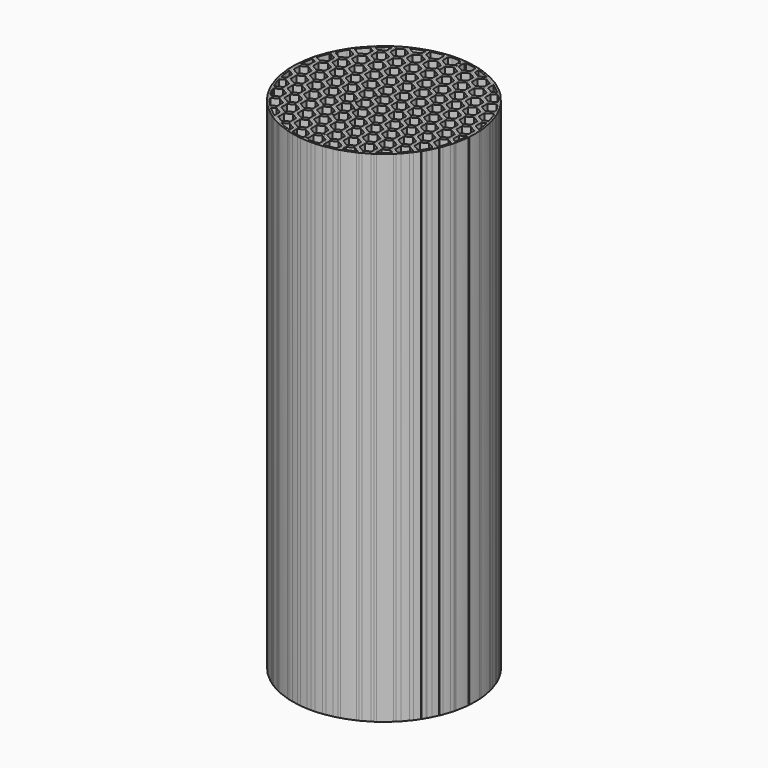
from build123d import *

# Parameters (mm, degrees)
F1_DEPTH  = 130
F0_R      = 23.75
F0_R_2    = 23.25
F14_R     = 45.818739932
F14_R_2   = 23.75
F15_DEPTH = 130


with BuildPart() as f1:
    # F0 (on Top) → F1 (new body)
    with BuildSketch(Plane.XY):
        Polygon((2.1135, -1.2202297939), (2.1135, 1.2202297939), (0, 2.4404595879), (-2.1135, 1.2202297939), (-2.1135, -1.2202297939), (0, -2.4404595879), align=None)
        Polygon((0, 1.8631093187), (1.6135, 0.9315546593), (1.6135, -0.9315546593), (0, -1.8631093187), (-1.6135, -0.9315546593), (-1.6135, 0.9315546593), align=None, mode=Mode.SUBTRACT)
    extrude(amount=F1_DEPTH)


with BuildPart() as f1b:
    # F0 (on Top) → F1, piece 2 (new body)
    with BuildSketch(Plane.XY):
        Circle(F0_R)
        Circle(F0_R_2, mode=Mode.SUBTRACT)
    extrude(amount=F1_DEPTH)


with BuildPart() as f3_1:
    # F3: copy of F1
    add(f1.part.moved(Location((4.227, 0, 0))))


with BuildPart() as f4_1:
    # F4: copy of F1
    add(f1.part.moved(Location((8.454, 0, 0))))


with BuildPart() as f4_2:
    # F4: copy of F3_1
    add(f3_1.part.moved(Location((8.454, 0, 0))))


with BuildPart() as f5_1:
    # F5: copy of F4_1
    add(f4_1.part.moved(Location((8.454, 0, 0))))


with BuildPart() as f5_2:
    # F5: copy of F4_2
    add(f4_2.part.moved(Location((8.454, 0, 0))))


with BuildPart() as f6_1:
    # F6: copy of F1
    add(f1.part.moved(Location((2.1135, 3.65, 0))))


with BuildPart() as f6_2:
    # F6: copy of F3_1
    add(f3_1.part.moved(Location((2.1135, 3.65, 0))))


with BuildPart() as f6_3:
    # F6: copy of F4_1
    add(f4_1.part.moved(Location((2.1135, 3.65, 0))))


with BuildPart() as f6_4:
    # F6: copy of F4_2
    add(f4_2.part.moved(Location((2.1135, 3.65, 0))))


with BuildPart() as f6_5:
    # F6: copy of F5_1
    add(f5_1.part.moved(Location((2.1135, 3.65, 0))))


with BuildPart() as f6_6:
    # F6: copy of F5_2
    add(f5_2.part.moved(Location((2.1135, 3.65, 0))))


with BuildPart() as f7_1:
    # F7: copy of F6_1
    add(f6_1.part.moved(Location((4.228, 7.3, 0))))


with BuildPart() as f7_2:
    # F7: copy of F1
    add(f1.part.moved(Location((4.228, 7.3, 0))))


with BuildPart() as f7_3:
    # F7: copy of F3_1
    add(f3_1.part.moved(Location((4.228, 7.3, 0))))


with BuildPart() as f7_4:
    # F7: copy of F6_2
    add(f6_2.part.moved(Location((4.228, 7.3, 0))))


with BuildPart() as f7_5:
    # F7: copy of F6_3
    add(f6_3.part.moved(Location((4.228, 7.3, 0))))


with BuildPart() as f7_6:
    # F7: copy of F4_1
    add(f4_1.part.moved(Location((4.228, 7.3, 0))))


with BuildPart() as f7_7:
    # F7: copy of F4_2
    add(f4_2.part.moved(Location((4.228, 7.3, 0))))


with BuildPart() as f7_8:
    # F7: copy of F6_4
    add(f6_4.part.moved(Location((4.228, 7.3, 0))))


with BuildPart() as f7_9:
    # F7: copy of F6_5
    add(f6_5.part.moved(Location((4.228, 7.3, 0))))


with BuildPart() as f7_10:
    # F7: copy of F5_1
    add(f5_1.part.moved(Location((4.228, 7.3, 0))))


with BuildPart() as f7_11:
    # F7: copy of F6_6
    add(f6_6.part.moved(Location((4.228, 7.3, 0))))


with BuildPart() as f7_12:
    # F7: copy of F5_2
    add(f5_2.part.moved(Location((4.228, 7.3, 0))))


with BuildPart() as f8_1:
    # F8: copy of F1
    add(f1.part.moved(Location((-4.228, -14.6, 0))))


with BuildPart() as f8_2:
    # F8: copy of F7_4
    add(f7_4.part.moved(Location((-4.228, -14.6, 0))))


with BuildPart() as f8_3:
    # F8: copy of F7_1
    add(f7_1.part.moved(Location((-4.228, -14.6, 0))))


with BuildPart() as f8_4:
    # F8: copy of F7_6
    add(f7_6.part.moved(Location((-4.228, -14.6, 0))))


with BuildPart() as f8_5:
    # F8: copy of F7_3
    add(f7_3.part.moved(Location((-4.228, -14.6, 0))))


with BuildPart() as f8_6:
    # F8: copy of F7_2
    add(f7_2.part.moved(Location((-4.228, -14.6, 0))))


with BuildPart() as f8_7:
    # F8: copy of F6_3
    add(f6_3.part.moved(Location((-4.228, -14.6, 0))))


with BuildPart() as f8_8:
    # F8: copy of F6_2
    add(f6_2.part.moved(Location((-4.228, -14.6, 0))))


with BuildPart() as f8_9:
    # F8: copy of F6_1
    add(f6_1.part.moved(Location((-4.228, -14.6, 0))))


with BuildPart() as f8_10:
    # F8: copy of F4_2
    add(f4_2.part.moved(Location((-4.228, -14.6, 0))))


with BuildPart() as f8_11:
    # F8: copy of F4_1
    add(f4_1.part.moved(Location((-4.228, -14.6, 0))))


with BuildPart() as f8_12:
    # F8: copy of F3_1
    add(f3_1.part.moved(Location((-4.228, -14.6, 0))))


with BuildPart() as f8_13:
    # F8: copy of F6_4
    add(f6_4.part.moved(Location((-4.228, -14.6, 0))))


with BuildPart() as f8_14:
    # F8: copy of F7_7
    add(f7_7.part.moved(Location((-4.228, -14.6, 0))))


with BuildPart() as f8_15:
    # F8: copy of F7_5
    add(f7_5.part.moved(Location((-4.228, -14.6, 0))))


with BuildPart() as f8_16:
    # F8: copy of F7_8
    add(f7_8.part.moved(Location((-4.228, -14.6, 0))))


with BuildPart() as f8_17:
    # F8: copy of F7_10
    add(f7_10.part.moved(Location((-4.228, -14.6, 0))))


with BuildPart() as f8_18:
    # F8: copy of F6_5
    add(f6_5.part.moved(Location((-4.228, -14.6, 0))))


with BuildPart() as f8_19:
    # F8: copy of F5_1
    add(f5_1.part.moved(Location((-4.228, -14.6, 0))))


with BuildPart() as f8_20:
    # F8: copy of F5_2
    add(f5_2.part.moved(Location((-4.228, -14.6, 0))))


with BuildPart() as f8_21:
    # F8: copy of F6_6
    add(f6_6.part.moved(Location((-4.228, -14.6, 0))))


with BuildPart() as f8_22:
    # F8: copy of F7_12
    add(f7_12.part.moved(Location((-4.228, -14.6, 0))))


with BuildPart() as f8_23:
    # F8: copy of F7_9
    add(f7_9.part.moved(Location((-4.228, -14.6, 0))))


with BuildPart() as f9_1:
    # F9: copy of F8_9
    add(f8_9.part.moved(Location((-25.369, 0, 0))))


with BuildPart() as f9_2:
    # F9: copy of F1
    add(f1.part.moved(Location((-25.369, 0, 0))))


with BuildPart() as f9_3:
    # F9: copy of F8_8
    add(f8_8.part.moved(Location((-25.369, 0, 0))))


with BuildPart() as f9_4:
    # F9: copy of F8_4
    add(f8_4.part.moved(Location((-25.369, 0, 0))))


with BuildPart() as f9_5:
    # F9: copy of F7_4
    add(f7_4.part.moved(Location((-25.369, 0, 0))))


with BuildPart() as f9_6:
    # F9: copy of F8_5
    add(f8_5.part.moved(Location((-25.369, 0, 0))))


with BuildPart() as f9_7:
    # F9: copy of F8_13
    add(f8_13.part.moved(Location((-25.369, 0, 0))))


with BuildPart() as f9_8:
    # F9: copy of F8_6
    add(f8_6.part.moved(Location((-25.369, 0, 0))))


with BuildPart() as f9_9:
    # F9: copy of F8_3
    add(f8_3.part.moved(Location((-25.369, 0, 0))))


with BuildPart() as f9_10:
    # F9: copy of F7_1
    add(f7_1.part.moved(Location((-25.369, 0, 0))))


with BuildPart() as f9_11:
    # F9: copy of F7_3
    add(f7_3.part.moved(Location((-25.369, 0, 0))))


with BuildPart() as f9_12:
    # F9: copy of F7_2
    add(f7_2.part.moved(Location((-25.369, 0, 0))))


with BuildPart() as f9_13:
    # F9: copy of F6_3
    add(f6_3.part.moved(Location((-25.369, 0, 0))))


with BuildPart() as f9_14:
    # F9: copy of F6_2
    add(f6_2.part.moved(Location((-25.369, 0, 0))))


with BuildPart() as f9_15:
    # F9: copy of F6_1
    add(f6_1.part.moved(Location((-25.369, 0, 0))))


with BuildPart() as f9_16:
    # F9: copy of F4_1
    add(f4_1.part.moved(Location((-25.369, 0, 0))))


with BuildPart() as f9_17:
    # F9: copy of F3_1
    add(f3_1.part.moved(Location((-25.369, 0, 0))))


with BuildPart() as f9_18:
    # F9: copy of F8_2
    add(f8_2.part.moved(Location((-25.369, 0, 0))))


with BuildPart() as f9_19:
    # F9: copy of F8_7
    add(f8_7.part.moved(Location((-25.369, 0, 0))))


with BuildPart() as f9_20:
    # F9: copy of F8_15
    add(f8_15.part.moved(Location((-25.369, 0, 0))))


with BuildPart() as f9_21:
    # F9: copy of F8_1
    add(f8_1.part.moved(Location((-25.369, 0, 0))))


with BuildPart() as f9_22:
    # F9: copy of F8_12
    add(f8_12.part.moved(Location((-25.369, 0, 0))))


with BuildPart() as f9_23:
    # F9: copy of F8_11
    add(f8_11.part.moved(Location((-25.369, 0, 0))))


with BuildPart() as f9_24:
    # F9: copy of F8_10
    add(f8_10.part.moved(Location((-25.369, 0, 0))))


with BuildPart() as f9_25:
    # F9: copy of F8_20
    add(f8_20.part.moved(Location((-25.369, 0, 0))))


with BuildPart() as f9_26:
    # F9: copy of F7_11
    add(f7_11.part.moved(Location((-25.369, 0, 0))))


with BuildPart() as f9_27:
    # F9: copy of F8_14
    add(f8_14.part.moved(Location((-25.369, 0, 0))))


with BuildPart() as f9_28:
    # F9: copy of F7_5
    add(f7_5.part.moved(Location((-25.369, 0, 0))))


with BuildPart() as f9_29:
    # F9: copy of F7_8
    add(f7_8.part.moved(Location((-25.369, 0, 0))))


with BuildPart() as f9_30:
    # F9: copy of F7_9
    add(f7_9.part.moved(Location((-25.369, 0, 0))))


with BuildPart() as f9_31:
    # F9: copy of F8_21
    add(f8_21.part.moved(Location((-25.369, 0, 0))))


with BuildPart() as f9_32:
    # F9: copy of F7_10
    add(f7_10.part.moved(Location((-25.369, 0, 0))))


with BuildPart() as f9_33:
    # F9: copy of F7_7
    add(f7_7.part.moved(Location((-25.369, 0, 0))))


with BuildPart() as f9_34:
    # F9: copy of F8_19
    add(f8_19.part.moved(Location((-25.369, 0, 0))))


with BuildPart() as f9_35:
    # F9: copy of F7_12
    add(f7_12.part.moved(Location((-25.369, 0, 0))))


with BuildPart() as f9_36:
    # F9: copy of F7_6
    add(f7_6.part.moved(Location((-25.369, 0, 0))))


with BuildPart() as f9_37:
    # F9: copy of F6_4
    add(f6_4.part.moved(Location((-25.369, 0, 0))))


with BuildPart() as f9_38:
    # F9: copy of F6_5
    add(f6_5.part.moved(Location((-25.369, 0, 0))))


with BuildPart() as f9_39:
    # F9: copy of F6_6
    add(f6_6.part.moved(Location((-25.369, 0, 0))))


with BuildPart() as f9_40:
    # F9: copy of F4_2
    add(f4_2.part.moved(Location((-25.369, 0, 0))))


with BuildPart() as f9_41:
    # F9: copy of F5_2
    add(f5_2.part.moved(Location((-25.369, 0, 0))))


with BuildPart() as f9_42:
    # F9: copy of F5_1
    add(f5_1.part.moved(Location((-25.369, 0, 0))))


with BuildPart() as f9_43:
    # F9: copy of F8_18
    add(f8_18.part.moved(Location((-25.369, 0, 0))))


with BuildPart() as f9_44:
    # F9: copy of F8_17
    add(f8_17.part.moved(Location((-25.369, 0, 0))))


with BuildPart() as f9_45:
    # F9: copy of F8_22
    add(f8_22.part.moved(Location((-25.369, 0, 0))))


with BuildPart() as f9_46:
    # F9: copy of F8_16
    add(f8_16.part.moved(Location((-25.369, 0, 0))))


with BuildPart() as f9_47:
    # F9: copy of F8_23
    add(f8_23.part.moved(Location((-25.369, 0, 0))))


with BuildPart() as f10_1:
    # F10: copy of F9_47
    add(f9_47.part.moved(Location((4.228, 0, 0))))


with BuildPart() as f11_1:
    # F11: copy of F8_1
    add(f8_1.part.moved(Location((0, -14.6, 0))))


with BuildPart() as f11_2:
    # F11: copy of F8_9
    add(f8_9.part.moved(Location((0, -14.6, 0))))


with BuildPart() as f11_3:
    # F11: copy of F8_8
    add(f8_8.part.moved(Location((0, -14.6, 0))))


with BuildPart() as f11_4:
    # F11: copy of F8_20
    add(f8_20.part.moved(Location((0, -14.6, 0))))


with BuildPart() as f11_5:
    # F11: copy of F8_4
    add(f8_4.part.moved(Location((0, -14.6, 0))))


with BuildPart() as f11_6:
    # F11: copy of F8_14
    add(f8_14.part.moved(Location((0, -14.6, 0))))


with BuildPart() as f11_7:
    # F11: copy of F8_5
    add(f8_5.part.moved(Location((0, -14.6, 0))))


with BuildPart() as f11_8:
    # F11: copy of F8_13
    add(f8_13.part.moved(Location((0, -14.6, 0))))


with BuildPart() as f11_9:
    # F11: copy of F8_21
    add(f8_21.part.moved(Location((0, -14.6, 0))))


with BuildPart() as f11_10:
    # F11: copy of F8_6
    add(f8_6.part.moved(Location((0, -14.6, 0))))


with BuildPart() as f11_11:
    # F11: copy of F8_19
    add(f8_19.part.moved(Location((0, -14.6, 0))))


with BuildPart() as f11_12:
    # F11: copy of F8_12
    add(f8_12.part.moved(Location((0, -14.6, 0))))


with BuildPart() as f11_13:
    # F11: copy of F8_11
    add(f8_11.part.moved(Location((0, -14.6, 0))))


with BuildPart() as f11_14:
    # F11: copy of F8_10
    add(f8_10.part.moved(Location((0, -14.6, 0))))


with BuildPart() as f11_15:
    # F11: copy of F8_18
    add(f8_18.part.moved(Location((0, -14.6, 0))))


with BuildPart() as f11_16:
    # F11: copy of F8_7
    add(f8_7.part.moved(Location((0, -14.6, 0))))


with BuildPart() as f11_17:
    # F11: copy of F8_17
    add(f8_17.part.moved(Location((0, -14.6, 0))))


with BuildPart() as f11_18:
    # F11: copy of F8_22
    add(f8_22.part.moved(Location((0, -14.6, 0))))


with BuildPart() as f11_19:
    # F11: copy of F9_21
    add(f9_21.part.moved(Location((0, -14.6, 0))))


with BuildPart() as f11_20:
    # F11: copy of F9_22
    add(f9_22.part.moved(Location((0, -14.6, 0))))


with BuildPart() as f11_21:
    # F11: copy of F9_23
    add(f9_23.part.moved(Location((0, -14.6, 0))))


with BuildPart() as f11_22:
    # F11: copy of F9_24
    add(f9_24.part.moved(Location((0, -14.6, 0))))


with BuildPart() as f11_23:
    # F11: copy of F9_34
    add(f9_34.part.moved(Location((0, -14.6, 0))))


with BuildPart() as f11_24:
    # F11: copy of F9_25
    add(f9_25.part.moved(Location((0, -14.6, 0))))


with BuildPart() as f11_25:
    # F11: copy of F9_1
    add(f9_1.part.moved(Location((0, -14.6, 0))))


with BuildPart() as f11_26:
    # F11: copy of F9_3
    add(f9_3.part.moved(Location((0, -14.6, 0))))


with BuildPart() as f11_27:
    # F11: copy of F9_19
    add(f9_19.part.moved(Location((0, -14.6, 0))))


with BuildPart() as f11_28:
    # F11: copy of F9_7
    add(f9_7.part.moved(Location((0, -14.6, 0))))


with BuildPart() as f11_29:
    # F11: copy of F9_43
    add(f9_43.part.moved(Location((0, -14.6, 0))))


with BuildPart() as f11_30:
    # F11: copy of F9_31
    add(f9_31.part.moved(Location((0, -14.6, 0))))


with BuildPart() as f11_31:
    # F11: copy of F9_8
    add(f9_8.part.moved(Location((0, -14.6, 0))))


with BuildPart() as f11_32:
    # F11: copy of F9_6
    add(f9_6.part.moved(Location((0, -14.6, 0))))


with BuildPart() as f11_33:
    # F11: copy of F9_4
    add(f9_4.part.moved(Location((0, -14.6, 0))))


with BuildPart() as f11_34:
    # F11: copy of F9_27
    add(f9_27.part.moved(Location((0, -14.6, 0))))


with BuildPart() as f11_35:
    # F11: copy of F9_44
    add(f9_44.part.moved(Location((0, -14.6, 0))))


with BuildPart() as f11_36:
    # F11: copy of F9_45
    add(f9_45.part.moved(Location((0, -14.6, 0))))


with BuildPart() as f11_37:
    # F11: copy of F8_3
    add(f8_3.part.moved(Location((0, -14.6, 0))))


with BuildPart() as f11_38:
    # F11: copy of F8_2
    add(f8_2.part.moved(Location((0, -14.6, 0))))


with BuildPart() as f11_39:
    # F11: copy of F8_15
    add(f8_15.part.moved(Location((0, -14.6, 0))))


with BuildPart() as f11_40:
    # F11: copy of F8_16
    add(f8_16.part.moved(Location((0, -14.6, 0))))


with BuildPart() as f11_41:
    # F11: copy of F8_23
    add(f8_23.part.moved(Location((0, -14.6, 0))))


with BuildPart() as f11_42:
    # F11: copy of F9_9
    add(f9_9.part.moved(Location((0, -14.6, 0))))


with BuildPart() as f11_43:
    # F11: copy of F9_18
    add(f9_18.part.moved(Location((0, -14.6, 0))))


with BuildPart() as f11_44:
    # F11: copy of F9_20
    add(f9_20.part.moved(Location((0, -14.6, 0))))


with BuildPart() as f11_45:
    # F11: copy of F9_46
    add(f9_46.part.moved(Location((0, -14.6, 0))))


with BuildPart() as f11_46:
    # F11: copy of F9_47
    add(f9_47.part.moved(Location((0, -14.6, 0))))


with BuildPart() as f11_47:
    # F11: copy of F10_1
    add(f10_1.part.moved(Location((0, -14.6, 0))))


with BuildPart() as f12_1:
    # F12: copy of F7_11
    add(f7_11.part.moved(Location((0, 14.6, 0))))


with BuildPart() as f12_2:
    # F12: copy of F7_4
    add(f7_4.part.moved(Location((0, 14.6, 0))))


with BuildPart() as f12_3:
    # F12: copy of F7_5
    add(f7_5.part.moved(Location((0, 14.6, 0))))


with BuildPart() as f12_4:
    # F12: copy of F7_8
    add(f7_8.part.moved(Location((0, 14.6, 0))))


with BuildPart() as f12_5:
    # F12: copy of F7_9
    add(f7_9.part.moved(Location((0, 14.6, 0))))


with BuildPart() as f12_6:
    # F12: copy of F7_10
    add(f7_10.part.moved(Location((0, 14.6, 0))))


with BuildPart() as f12_7:
    # F12: copy of F7_7
    add(f7_7.part.moved(Location((0, 14.6, 0))))


with BuildPart() as f12_8:
    # F12: copy of F7_12
    add(f7_12.part.moved(Location((0, 14.6, 0))))


with BuildPart() as f12_9:
    # F12: copy of F7_1
    add(f7_1.part.moved(Location((0, 14.6, 0))))


with BuildPart() as f12_10:
    # F12: copy of F7_6
    add(f7_6.part.moved(Location((0, 14.6, 0))))


with BuildPart() as f12_11:
    # F12: copy of F7_3
    add(f7_3.part.moved(Location((0, 14.6, 0))))


with BuildPart() as f12_12:
    # F12: copy of F7_2
    add(f7_2.part.moved(Location((0, 14.6, 0))))


with BuildPart() as f12_13:
    # F12: copy of F9_12
    add(f9_12.part.moved(Location((0, 14.6, 0))))


with BuildPart() as f12_14:
    # F12: copy of F9_11
    add(f9_11.part.moved(Location((0, 14.6, 0))))


with BuildPart() as f12_15:
    # F12: copy of F9_36
    add(f9_36.part.moved(Location((0, 14.6, 0))))


with BuildPart() as f12_16:
    # F12: copy of F9_33
    add(f9_33.part.moved(Location((0, 14.6, 0))))


with BuildPart() as f12_17:
    # F12: copy of F9_32
    add(f9_32.part.moved(Location((0, 14.6, 0))))


with BuildPart() as f12_18:
    # F12: copy of F9_35
    add(f9_35.part.moved(Location((0, 14.6, 0))))


with BuildPart() as f12_19:
    # F12: copy of F9_10
    add(f9_10.part.moved(Location((0, 14.6, 0))))


with BuildPart() as f12_20:
    # F12: copy of F9_5
    add(f9_5.part.moved(Location((0, 14.6, 0))))


with BuildPart() as f12_21:
    # F12: copy of F9_28
    add(f9_28.part.moved(Location((0, 14.6, 0))))


with BuildPart() as f12_22:
    # F12: copy of F9_29
    add(f9_29.part.moved(Location((0, 14.6, 0))))


with BuildPart() as f12_23:
    # F12: copy of F9_30
    add(f9_30.part.moved(Location((0, 14.6, 0))))


with BuildPart() as f12_24:
    # F12: copy of F9_26
    add(f9_26.part.moved(Location((0, 14.6, 0))))


with BuildPart() as f12_25:
    # F12: copy of F9_15
    add(f9_15.part.moved(Location((0, 14.6, 0))))


with BuildPart() as f12_26:
    # F12: copy of F9_14
    add(f9_14.part.moved(Location((0, 14.6, 0))))


with BuildPart() as f12_27:
    # F12: copy of F9_13
    add(f9_13.part.moved(Location((0, 14.6, 0))))


with BuildPart() as f12_28:
    # F12: copy of F9_37
    add(f9_37.part.moved(Location((0, 14.6, 0))))


with BuildPart() as f12_29:
    # F12: copy of F9_38
    add(f9_38.part.moved(Location((0, 14.6, 0))))


with BuildPart() as f12_30:
    # F12: copy of F9_39
    add(f9_39.part.moved(Location((0, 14.6, 0))))


with BuildPart() as f12_31:
    # F12: copy of F6_1
    add(f6_1.part.moved(Location((0, 14.6, 0))))


with BuildPart() as f12_32:
    # F12: copy of F6_2
    add(f6_2.part.moved(Location((0, 14.6, 0))))


with BuildPart() as f12_33:
    # F12: copy of F6_3
    add(f6_3.part.moved(Location((0, 14.6, 0))))


with BuildPart() as f12_34:
    # F12: copy of F1
    add(f1.part.moved(Location((0, 14.6, 0))))


with BuildPart() as f12_35:
    # F12: copy of F6_4
    add(f6_4.part.moved(Location((0, 14.6, 0))))


with BuildPart() as f12_36:
    # F12: copy of F6_5
    add(f6_5.part.moved(Location((0, 14.6, 0))))


with BuildPart() as f12_37:
    # F12: copy of F6_6
    add(f6_6.part.moved(Location((0, 14.6, 0))))


with BuildPart() as f12_38:
    # F12: copy of F4_2
    add(f4_2.part.moved(Location((0, 14.6, 0))))


with BuildPart() as f12_39:
    # F12: copy of F5_2
    add(f5_2.part.moved(Location((0, 14.6, 0))))


with BuildPart() as f12_40:
    # F12: copy of F4_1
    add(f4_1.part.moved(Location((0, 14.6, 0))))


with BuildPart() as f12_41:
    # F12: copy of F5_1
    add(f5_1.part.moved(Location((0, 14.6, 0))))


with BuildPart() as f12_42:
    # F12: copy of F3_1
    add(f3_1.part.moved(Location((0, 14.6, 0))))


with BuildPart() as f12_43:
    # F12: copy of F9_2
    add(f9_2.part.moved(Location((0, 14.6, 0))))


with BuildPart() as f12_44:
    # F12: copy of F9_17
    add(f9_17.part.moved(Location((0, 14.6, 0))))


with BuildPart() as f12_45:
    # F12: copy of F9_16
    add(f9_16.part.moved(Location((0, 14.6, 0))))


with BuildPart() as f12_46:
    # F12: copy of F9_40
    add(f9_40.part.moved(Location((0, 14.6, 0))))


with BuildPart() as f12_47:
    # F12: copy of F9_42
    add(f9_42.part.moved(Location((0, 14.6, 0))))


with BuildPart() as f12_48:
    # F12: copy of F9_41
    add(f9_41.part.moved(Location((0, 14.6, 0))))


with BuildPart() as f13_1:
    # F13: copy of F8_23
    add(f8_23.part.moved(Location((4.228, 0, 0))))


with BuildPart() as f15:
    # F14 (on Top) → F15 (new body)
    with BuildSketch(Plane.XY):
        Circle(F14_R)
        Circle(F14_R_2, mode=Mode.SUBTRACT)
    extrude(amount=F15_DEPTH)


with BuildPart() as f12_5_1:
    add(f12_5.part)

    # F16: cut F15
    add(f15.part, mode=Mode.SUBTRACT)


with BuildPart() as f12_6_1:
    add(f12_6.part)

    # F16: cut F15
    add(f15.part, mode=Mode.SUBTRACT)


with BuildPart() as f1b_1:
    add(f1b.part)

    # F16: cut F15
    add(f15.part, mode=Mode.SUBTRACT)


with BuildPart() as f12_7_1:
    add(f12_7.part)

    # F16: cut F15
    add(f15.part, mode=Mode.SUBTRACT)


with BuildPart() as f12_8_1:
    add(f12_8.part)

    # F16: cut F15
    add(f15.part, mode=Mode.SUBTRACT)


with BuildPart() as f12_1_1:
    add(f12_1.part)

    # F16: cut F15
    add(f15.part, mode=Mode.SUBTRACT)


with BuildPart() as f12_33_1:
    add(f12_33.part)

    # F16: cut F15
    add(f15.part, mode=Mode.SUBTRACT)


with BuildPart() as f12_46_1:
    add(f12_46.part)

    # F16: cut F15
    add(f15.part, mode=Mode.SUBTRACT)


with BuildPart() as f12_32_1:
    add(f12_32.part)

    # F16: cut F15
    add(f15.part, mode=Mode.SUBTRACT)


with BuildPart() as f12_35_1:
    add(f12_35.part)

    # F16: cut F15
    add(f15.part, mode=Mode.SUBTRACT)


with BuildPart() as f12_45_1:
    add(f12_45.part)

    # F16: cut F15
    add(f15.part, mode=Mode.SUBTRACT)


with BuildPart() as f12_44_1:
    add(f12_44.part)

    # F16: cut F15
    add(f15.part, mode=Mode.SUBTRACT)


with BuildPart() as f12_43_1:
    add(f12_43.part)

    # F16: cut F15
    add(f15.part, mode=Mode.SUBTRACT)


with BuildPart() as f12_11_1:
    add(f12_11.part)

    # F16: cut F15
    add(f15.part, mode=Mode.SUBTRACT)


with BuildPart() as f12_37_1:
    add(f12_37.part)

    # F16: cut F15
    add(f15.part, mode=Mode.SUBTRACT)


with BuildPart() as f12_36_1:
    add(f12_36.part)

    # F16: cut F15
    add(f15.part, mode=Mode.SUBTRACT)


with BuildPart() as f12_25_1:
    add(f12_25.part)

    # F16: cut F15
    add(f15.part, mode=Mode.SUBTRACT)


with BuildPart() as f12_41_1:
    add(f12_41.part)

    # F16: cut F15
    add(f15.part, mode=Mode.SUBTRACT)


with BuildPart() as f12_26_1:
    add(f12_26.part)

    # F16: cut F15
    add(f15.part, mode=Mode.SUBTRACT)


with BuildPart() as f12_9_1:
    add(f12_9.part)

    # F16: cut F15
    add(f15.part, mode=Mode.SUBTRACT)


with BuildPart() as f12_4_1:
    add(f12_4.part)

    # F16: cut F15
    add(f15.part, mode=Mode.SUBTRACT)


with BuildPart() as f12_3_1:
    add(f12_3.part)

    # F16: cut F15
    add(f15.part, mode=Mode.SUBTRACT)


with BuildPart() as f12_2_1:
    add(f12_2.part)

    # F16: cut F15
    add(f15.part, mode=Mode.SUBTRACT)


with BuildPart() as f12_48_1:
    add(f12_48.part)

    # F16: cut F15
    add(f15.part, mode=Mode.SUBTRACT)


with BuildPart() as f12_47_1:
    add(f12_47.part)

    # F16: cut F15
    add(f15.part, mode=Mode.SUBTRACT)


with BuildPart() as f12_27_1:
    add(f12_27.part)

    # F16: cut F15
    add(f15.part, mode=Mode.SUBTRACT)


with BuildPart() as f12_28_1:
    add(f12_28.part)

    # F16: cut F15
    add(f15.part, mode=Mode.SUBTRACT)


with BuildPart() as f12_29_1:
    add(f12_29.part)

    # F16: cut F15
    add(f15.part, mode=Mode.SUBTRACT)


with BuildPart() as f12_14_1:
    add(f12_14.part)

    # F16: cut F15
    add(f15.part, mode=Mode.SUBTRACT)


with BuildPart() as f12_13_1:
    add(f12_13.part)

    # F16: cut F15
    add(f15.part, mode=Mode.SUBTRACT)


with BuildPart() as f12_30_1:
    add(f12_30.part)

    # F16: cut F15
    add(f15.part, mode=Mode.SUBTRACT)


with BuildPart() as f12_15_1:
    add(f12_15.part)

    # F16: cut F15
    add(f15.part, mode=Mode.SUBTRACT)


with BuildPart() as f12_16_1:
    add(f12_16.part)

    # F16: cut F15
    add(f15.part, mode=Mode.SUBTRACT)


with BuildPart() as f12_17_1:
    add(f12_17.part)

    # F16: cut F15
    add(f15.part, mode=Mode.SUBTRACT)


with BuildPart() as f12_20_1:
    add(f12_20.part)

    # F16: cut F15
    add(f15.part, mode=Mode.SUBTRACT)


with BuildPart() as f12_18_1:
    add(f12_18.part)

    # F16: cut F15
    add(f15.part, mode=Mode.SUBTRACT)


with BuildPart() as f12_23_1:
    add(f12_23.part)

    # F16: cut F15
    add(f15.part, mode=Mode.SUBTRACT)


with BuildPart() as f12_21_1:
    add(f12_21.part)

    # F16: cut F15
    add(f15.part, mode=Mode.SUBTRACT)


with BuildPart() as f12_19_1:
    add(f12_19.part)

    # F16: cut F15
    add(f15.part, mode=Mode.SUBTRACT)


with BuildPart() as f12_22_1:
    add(f12_22.part)

    # F16: cut F15
    add(f15.part, mode=Mode.SUBTRACT)


with BuildPart() as f12_24_1:
    add(f12_24.part)

    # F16: cut F15
    add(f15.part, mode=Mode.SUBTRACT)


with BuildPart() as f12_38_1:
    add(f12_38.part)

    # F16: cut F15
    add(f15.part, mode=Mode.SUBTRACT)


with BuildPart() as f12_12_1:
    add(f12_12.part)

    # F16: cut F15
    add(f15.part, mode=Mode.SUBTRACT)


with BuildPart() as f12_10_1:
    add(f12_10.part)

    # F16: cut F15
    add(f15.part, mode=Mode.SUBTRACT)


with BuildPart() as f12_31_1:
    add(f12_31.part)

    # F16: cut F15
    add(f15.part, mode=Mode.SUBTRACT)


with BuildPart() as f12_39_1:
    add(f12_39.part)

    # F16: cut F15
    add(f15.part, mode=Mode.SUBTRACT)


with BuildPart() as f12_40_1:
    add(f12_40.part)

    # F16: cut F15
    add(f15.part, mode=Mode.SUBTRACT)


with BuildPart() as f12_42_1:
    add(f12_42.part)

    # F16: cut F15
    add(f15.part, mode=Mode.SUBTRACT)


with BuildPart() as f12_34_1:
    add(f12_34.part)

    # F16: cut F15
    add(f15.part, mode=Mode.SUBTRACT)


with BuildPart() as f11_47_1:
    add(f11_47.part)

    # F16: cut F15
    add(f15.part, mode=Mode.SUBTRACT)


with BuildPart() as f11_46_1:
    add(f11_46.part)

    # F16: cut F15
    add(f15.part, mode=Mode.SUBTRACT)


with BuildPart() as f11_45_1:
    add(f11_45.part)

    # F16: cut F15
    add(f15.part, mode=Mode.SUBTRACT)


with BuildPart() as f11_44_1:
    add(f11_44.part)

    # F16: cut F15
    add(f15.part, mode=Mode.SUBTRACT)


with BuildPart() as f11_43_1:
    add(f11_43.part)

    # F16: cut F15
    add(f15.part, mode=Mode.SUBTRACT)


with BuildPart() as f11_42_1:
    add(f11_42.part)

    # F16: cut F15
    add(f15.part, mode=Mode.SUBTRACT)


with BuildPart() as f11_36_1:
    add(f11_36.part)

    # F16: cut F15
    add(f15.part, mode=Mode.SUBTRACT)


with BuildPart() as f11_35_1:
    add(f11_35.part)

    # F16: cut F15
    add(f15.part, mode=Mode.SUBTRACT)


with BuildPart() as f11_34_1:
    add(f11_34.part)

    # F16: cut F15
    add(f15.part, mode=Mode.SUBTRACT)


with BuildPart() as f11_33_1:
    add(f11_33.part)

    # F16: cut F15
    add(f15.part, mode=Mode.SUBTRACT)


with BuildPart() as f11_32_1:
    add(f11_32.part)

    # F16: cut F15
    add(f15.part, mode=Mode.SUBTRACT)


with BuildPart() as f11_31_1:
    add(f11_31.part)

    # F16: cut F15
    add(f15.part, mode=Mode.SUBTRACT)


with BuildPart() as f11_30_1:
    add(f11_30.part)

    # F16: cut F15
    add(f15.part, mode=Mode.SUBTRACT)


with BuildPart() as f11_29_1:
    add(f11_29.part)

    # F16: cut F15
    add(f15.part, mode=Mode.SUBTRACT)


with BuildPart() as f11_28_1:
    add(f11_28.part)

    # F16: cut F15
    add(f15.part, mode=Mode.SUBTRACT)


with BuildPart() as f11_27_1:
    add(f11_27.part)

    # F16: cut F15
    add(f15.part, mode=Mode.SUBTRACT)


with BuildPart() as f11_26_1:
    add(f11_26.part)

    # F16: cut F15
    add(f15.part, mode=Mode.SUBTRACT)


with BuildPart() as f11_25_1:
    add(f11_25.part)

    # F16: cut F15
    add(f15.part, mode=Mode.SUBTRACT)


with BuildPart() as f11_24_1:
    add(f11_24.part)

    # F16: cut F15
    add(f15.part, mode=Mode.SUBTRACT)


with BuildPart() as f11_23_1:
    add(f11_23.part)

    # F16: cut F15
    add(f15.part, mode=Mode.SUBTRACT)


with BuildPart() as f11_22_1:
    add(f11_22.part)

    # F16: cut F15
    add(f15.part, mode=Mode.SUBTRACT)


with BuildPart() as f11_21_1:
    add(f11_21.part)

    # F16: cut F15
    add(f15.part, mode=Mode.SUBTRACT)


with BuildPart() as f11_20_1:
    add(f11_20.part)

    # F16: cut F15
    add(f15.part, mode=Mode.SUBTRACT)


with BuildPart() as f11_19_1:
    add(f11_19.part)

    # F16: cut F15
    add(f15.part, mode=Mode.SUBTRACT)


with BuildPart() as f11_41_1:
    add(f11_41.part)

    # F16: cut F15
    add(f15.part, mode=Mode.SUBTRACT)


with BuildPart() as f11_40_1:
    add(f11_40.part)

    # F16: cut F15
    add(f15.part, mode=Mode.SUBTRACT)


with BuildPart() as f11_39_1:
    add(f11_39.part)

    # F16: cut F15
    add(f15.part, mode=Mode.SUBTRACT)


with BuildPart() as f11_38_1:
    add(f11_38.part)

    # F16: cut F15
    add(f15.part, mode=Mode.SUBTRACT)


with BuildPart() as f11_37_1:
    add(f11_37.part)

    # F16: cut F15
    add(f15.part, mode=Mode.SUBTRACT)


with BuildPart() as f11_18_1:
    add(f11_18.part)

    # F16: cut F15
    add(f15.part, mode=Mode.SUBTRACT)


with BuildPart() as f11_17_1:
    add(f11_17.part)

    # F16: cut F15
    add(f15.part, mode=Mode.SUBTRACT)


with BuildPart() as f11_6_1:
    add(f11_6.part)

    # F16: cut F15
    add(f15.part, mode=Mode.SUBTRACT)


with BuildPart() as f11_5_1:
    add(f11_5.part)

    # F16: cut F15
    add(f15.part, mode=Mode.SUBTRACT)


with BuildPart() as f11_7_1:
    add(f11_7.part)

    # F16: cut F15
    add(f15.part, mode=Mode.SUBTRACT)


with BuildPart() as f11_10_1:
    add(f11_10.part)

    # F16: cut F15
    add(f15.part, mode=Mode.SUBTRACT)


with BuildPart() as f11_9_1:
    add(f11_9.part)

    # F16: cut F15
    add(f15.part, mode=Mode.SUBTRACT)


with BuildPart() as f11_15_1:
    add(f11_15.part)

    # F16: cut F15
    add(f15.part, mode=Mode.SUBTRACT)


with BuildPart() as f11_8_1:
    add(f11_8.part)

    # F16: cut F15
    add(f15.part, mode=Mode.SUBTRACT)


with BuildPart() as f11_16_1:
    add(f11_16.part)

    # F16: cut F15
    add(f15.part, mode=Mode.SUBTRACT)


with BuildPart() as f11_3_1:
    add(f11_3.part)

    # F16: cut F15
    add(f15.part, mode=Mode.SUBTRACT)


with BuildPart() as f11_2_1:
    add(f11_2.part)

    # F16: cut F15
    add(f15.part, mode=Mode.SUBTRACT)


with BuildPart() as f11_4_1:
    add(f11_4.part)

    # F16: cut F15
    add(f15.part, mode=Mode.SUBTRACT)


with BuildPart() as f11_11_1:
    add(f11_11.part)

    # F16: cut F15
    add(f15.part, mode=Mode.SUBTRACT)


with BuildPart() as f11_14_1:
    add(f11_14.part)

    # F16: cut F15
    add(f15.part, mode=Mode.SUBTRACT)


with BuildPart() as f11_13_1:
    add(f11_13.part)

    # F16: cut F15
    add(f15.part, mode=Mode.SUBTRACT)


with BuildPart() as f11_12_1:
    add(f11_12.part)

    # F16: cut F15
    add(f15.part, mode=Mode.SUBTRACT)


with BuildPart() as f11_1_1:
    add(f11_1.part)

    # F16: cut F15
    add(f15.part, mode=Mode.SUBTRACT)


with BuildPart() as f10_1_1:
    add(f10_1.part)

    # F16: cut F15
    add(f15.part, mode=Mode.SUBTRACT)


with BuildPart() as f9_47_1:
    add(f9_47.part)

    # F16: cut F15
    add(f15.part, mode=Mode.SUBTRACT)


with BuildPart() as f9_46_1:
    add(f9_46.part)

    # F16: cut F15
    add(f15.part, mode=Mode.SUBTRACT)


with BuildPart() as f9_20_1:
    add(f9_20.part)

    # F16: cut F15
    add(f15.part, mode=Mode.SUBTRACT)


with BuildPart() as f9_18_1:
    add(f9_18.part)

    # F16: cut F15
    add(f15.part, mode=Mode.SUBTRACT)


with BuildPart() as f9_9_1:
    add(f9_9.part)

    # F16: cut F15
    add(f15.part, mode=Mode.SUBTRACT)


with BuildPart() as f9_45_1:
    add(f9_45.part)

    # F16: cut F15
    add(f15.part, mode=Mode.SUBTRACT)


with BuildPart() as f9_44_1:
    add(f9_44.part)

    # F16: cut F15
    add(f15.part, mode=Mode.SUBTRACT)


with BuildPart() as f9_27_1:
    add(f9_27.part)

    # F16: cut F15
    add(f15.part, mode=Mode.SUBTRACT)


with BuildPart() as f9_4_1:
    add(f9_4.part)

    # F16: cut F15
    add(f15.part, mode=Mode.SUBTRACT)


with BuildPart() as f9_6_1:
    add(f9_6.part)

    # F16: cut F15
    add(f15.part, mode=Mode.SUBTRACT)


with BuildPart() as f9_8_1:
    add(f9_8.part)

    # F16: cut F15
    add(f15.part, mode=Mode.SUBTRACT)


with BuildPart() as f9_31_1:
    add(f9_31.part)

    # F16: cut F15
    add(f15.part, mode=Mode.SUBTRACT)


with BuildPart() as f9_43_1:
    add(f9_43.part)

    # F16: cut F15
    add(f15.part, mode=Mode.SUBTRACT)


with BuildPart() as f9_7_1:
    add(f9_7.part)

    # F16: cut F15
    add(f15.part, mode=Mode.SUBTRACT)


with BuildPart() as f9_19_1:
    add(f9_19.part)

    # F16: cut F15
    add(f15.part, mode=Mode.SUBTRACT)


with BuildPart() as f9_3_1:
    add(f9_3.part)

    # F16: cut F15
    add(f15.part, mode=Mode.SUBTRACT)


with BuildPart() as f9_1_1:
    add(f9_1.part)

    # F16: cut F15
    add(f15.part, mode=Mode.SUBTRACT)


with BuildPart() as f9_25_1:
    add(f9_25.part)

    # F16: cut F15
    add(f15.part, mode=Mode.SUBTRACT)


with BuildPart() as f9_34_1:
    add(f9_34.part)

    # F16: cut F15
    add(f15.part, mode=Mode.SUBTRACT)


with BuildPart() as f9_24_1:
    add(f9_24.part)

    # F16: cut F15
    add(f15.part, mode=Mode.SUBTRACT)


with BuildPart() as f9_23_1:
    add(f9_23.part)

    # F16: cut F15
    add(f15.part, mode=Mode.SUBTRACT)


with BuildPart() as f9_22_1:
    add(f9_22.part)

    # F16: cut F15
    add(f15.part, mode=Mode.SUBTRACT)


with BuildPart() as f9_21_1:
    add(f9_21.part)

    # F16: cut F15
    add(f15.part, mode=Mode.SUBTRACT)


with BuildPart() as f9_26_1:
    add(f9_26.part)

    # F16: cut F15
    add(f15.part, mode=Mode.SUBTRACT)


with BuildPart() as f9_30_1:
    add(f9_30.part)

    # F16: cut F15
    add(f15.part, mode=Mode.SUBTRACT)


with BuildPart() as f9_29_1:
    add(f9_29.part)

    # F16: cut F15
    add(f15.part, mode=Mode.SUBTRACT)


with BuildPart() as f9_28_1:
    add(f9_28.part)

    # F16: cut F15
    add(f15.part, mode=Mode.SUBTRACT)


with BuildPart() as f9_5_1:
    add(f9_5.part)

    # F16: cut F15
    add(f15.part, mode=Mode.SUBTRACT)


with BuildPart() as f9_10_1:
    add(f9_10.part)

    # F16: cut F15
    add(f15.part, mode=Mode.SUBTRACT)


with BuildPart() as f9_35_1:
    add(f9_35.part)

    # F16: cut F15
    add(f15.part, mode=Mode.SUBTRACT)


with BuildPart() as f9_32_1:
    add(f9_32.part)

    # F16: cut F15
    add(f15.part, mode=Mode.SUBTRACT)


with BuildPart() as f9_33_1:
    add(f9_33.part)

    # F16: cut F15
    add(f15.part, mode=Mode.SUBTRACT)


with BuildPart() as f9_36_1:
    add(f9_36.part)

    # F16: cut F15
    add(f15.part, mode=Mode.SUBTRACT)


with BuildPart() as f9_11_1:
    add(f9_11.part)

    # F16: cut F15
    add(f15.part, mode=Mode.SUBTRACT)


with BuildPart() as f9_12_1:
    add(f9_12.part)

    # F16: cut F15
    add(f15.part, mode=Mode.SUBTRACT)


with BuildPart() as f9_39_1:
    add(f9_39.part)

    # F16: cut F15
    add(f15.part, mode=Mode.SUBTRACT)


with BuildPart() as f9_38_1:
    add(f9_38.part)

    # F16: cut F15
    add(f15.part, mode=Mode.SUBTRACT)


with BuildPart() as f9_37_1:
    add(f9_37.part)

    # F16: cut F15
    add(f15.part, mode=Mode.SUBTRACT)


with BuildPart() as f9_13_1:
    add(f9_13.part)

    # F16: cut F15
    add(f15.part, mode=Mode.SUBTRACT)


with BuildPart() as f9_14_1:
    add(f9_14.part)

    # F16: cut F15
    add(f15.part, mode=Mode.SUBTRACT)


with BuildPart() as f9_15_1:
    add(f9_15.part)

    # F16: cut F15
    add(f15.part, mode=Mode.SUBTRACT)


with BuildPart() as f9_41_1:
    add(f9_41.part)

    # F16: cut F15
    add(f15.part, mode=Mode.SUBTRACT)


with BuildPart() as f9_42_1:
    add(f9_42.part)

    # F16: cut F15
    add(f15.part, mode=Mode.SUBTRACT)


with BuildPart() as f9_40_1:
    add(f9_40.part)

    # F16: cut F15
    add(f15.part, mode=Mode.SUBTRACT)


with BuildPart() as f9_16_1:
    add(f9_16.part)

    # F16: cut F15
    add(f15.part, mode=Mode.SUBTRACT)


with BuildPart() as f9_17_1:
    add(f9_17.part)

    # F16: cut F15
    add(f15.part, mode=Mode.SUBTRACT)


with BuildPart() as f9_2_1:
    add(f9_2.part)

    # F16: cut F15
    add(f15.part, mode=Mode.SUBTRACT)


with BuildPart() as f8_23_1:
    add(f8_23.part)

    # F16: cut F15
    add(f15.part, mode=Mode.SUBTRACT)


with BuildPart() as f8_16_1:
    add(f8_16.part)

    # F16: cut F15
    add(f15.part, mode=Mode.SUBTRACT)


with BuildPart() as f8_15_1:
    add(f8_15.part)

    # F16: cut F15
    add(f15.part, mode=Mode.SUBTRACT)


with BuildPart() as f8_2_1:
    add(f8_2.part)

    # F16: cut F15
    add(f15.part, mode=Mode.SUBTRACT)


with BuildPart() as f8_3_1:
    add(f8_3.part)

    # F16: cut F15
    add(f15.part, mode=Mode.SUBTRACT)


with BuildPart() as f8_22_1:
    add(f8_22.part)

    # F16: cut F15
    add(f15.part, mode=Mode.SUBTRACT)


with BuildPart() as f8_17_1:
    add(f8_17.part)

    # F16: cut F15
    add(f15.part, mode=Mode.SUBTRACT)


with BuildPart() as f8_14_1:
    add(f8_14.part)

    # F16: cut F15
    add(f15.part, mode=Mode.SUBTRACT)


with BuildPart() as f8_4_1:
    add(f8_4.part)

    # F16: cut F15
    add(f15.part, mode=Mode.SUBTRACT)


with BuildPart() as f8_5_1:
    add(f8_5.part)

    # F16: cut F15
    add(f15.part, mode=Mode.SUBTRACT)


with BuildPart() as f8_6_1:
    add(f8_6.part)

    # F16: cut F15
    add(f15.part, mode=Mode.SUBTRACT)


with BuildPart() as f8_21_1:
    add(f8_21.part)

    # F16: cut F15
    add(f15.part, mode=Mode.SUBTRACT)


with BuildPart() as f8_18_1:
    add(f8_18.part)

    # F16: cut F15
    add(f15.part, mode=Mode.SUBTRACT)


with BuildPart() as f8_13_1:
    add(f8_13.part)

    # F16: cut F15
    add(f15.part, mode=Mode.SUBTRACT)


with BuildPart() as f8_7_1:
    add(f8_7.part)

    # F16: cut F15
    add(f15.part, mode=Mode.SUBTRACT)


with BuildPart() as f8_8_1:
    add(f8_8.part)

    # F16: cut F15
    add(f15.part, mode=Mode.SUBTRACT)


with BuildPart() as f8_9_1:
    add(f8_9.part)

    # F16: cut F15
    add(f15.part, mode=Mode.SUBTRACT)


with BuildPart() as f8_20_1:
    add(f8_20.part)

    # F16: cut F15
    add(f15.part, mode=Mode.SUBTRACT)


with BuildPart() as f8_19_1:
    add(f8_19.part)

    # F16: cut F15
    add(f15.part, mode=Mode.SUBTRACT)


with BuildPart() as f8_10_1:
    add(f8_10.part)

    # F16: cut F15
    add(f15.part, mode=Mode.SUBTRACT)


with BuildPart() as f8_11_1:
    add(f8_11.part)

    # F16: cut F15
    add(f15.part, mode=Mode.SUBTRACT)


with BuildPart() as f8_12_1:
    add(f8_12.part)

    # F16: cut F15
    add(f15.part, mode=Mode.SUBTRACT)


with BuildPart() as f8_1_1:
    add(f8_1.part)

    # F16: cut F15
    add(f15.part, mode=Mode.SUBTRACT)


with BuildPart() as f7_11_1:
    add(f7_11.part)

    # F16: cut F15
    add(f15.part, mode=Mode.SUBTRACT)


with BuildPart() as f7_9_1:
    add(f7_9.part)

    # F16: cut F15
    add(f15.part, mode=Mode.SUBTRACT)


with BuildPart() as f7_8_1:
    add(f7_8.part)

    # F16: cut F15
    add(f15.part, mode=Mode.SUBTRACT)


with BuildPart() as f7_5_1:
    add(f7_5.part)

    # F16: cut F15
    add(f15.part, mode=Mode.SUBTRACT)


with BuildPart() as f7_4_1:
    add(f7_4.part)

    # F16: cut F15
    add(f15.part, mode=Mode.SUBTRACT)


with BuildPart() as f7_1_1:
    add(f7_1.part)

    # F16: cut F15
    add(f15.part, mode=Mode.SUBTRACT)


with BuildPart() as f7_12_1:
    add(f7_12.part)

    # F16: cut F15
    add(f15.part, mode=Mode.SUBTRACT)


with BuildPart() as f7_10_1:
    add(f7_10.part)

    # F16: cut F15
    add(f15.part, mode=Mode.SUBTRACT)


with BuildPart() as f7_7_1:
    add(f7_7.part)

    # F16: cut F15
    add(f15.part, mode=Mode.SUBTRACT)


with BuildPart() as f7_6_1:
    add(f7_6.part)

    # F16: cut F15
    add(f15.part, mode=Mode.SUBTRACT)


with BuildPart() as f7_3_1:
    add(f7_3.part)

    # F16: cut F15
    add(f15.part, mode=Mode.SUBTRACT)


with BuildPart() as f7_2_1:
    add(f7_2.part)

    # F16: cut F15
    add(f15.part, mode=Mode.SUBTRACT)


with BuildPart() as f6_6_1:
    add(f6_6.part)

    # F16: cut F15
    add(f15.part, mode=Mode.SUBTRACT)


with BuildPart() as f6_5_1:
    add(f6_5.part)

    # F16: cut F15
    add(f15.part, mode=Mode.SUBTRACT)


with BuildPart() as f6_4_1:
    add(f6_4.part)

    # F16: cut F15
    add(f15.part, mode=Mode.SUBTRACT)


with BuildPart() as f4_1_1:
    add(f4_1.part)

    # F16: cut F15
    add(f15.part, mode=Mode.SUBTRACT)


with BuildPart() as f4_2_1:
    add(f4_2.part)

    # F16: cut F15
    add(f15.part, mode=Mode.SUBTRACT)


with BuildPart() as f5_1_1:
    add(f5_1.part)

    # F16: cut F15
    add(f15.part, mode=Mode.SUBTRACT)


with BuildPart() as f5_2_1:
    add(f5_2.part)

    # F16: cut F15
    add(f15.part, mode=Mode.SUBTRACT)


with BuildPart() as f6_1_1:
    add(f6_1.part)

    # F16: cut F15
    add(f15.part, mode=Mode.SUBTRACT)


with BuildPart() as f6_2_1:
    add(f6_2.part)

    # F16: cut F15
    add(f15.part, mode=Mode.SUBTRACT)


with BuildPart() as f6_3_1:
    add(f6_3.part)

    # F16: cut F15
    add(f15.part, mode=Mode.SUBTRACT)


with BuildPart() as f3_1_1:
    add(f3_1.part)

    # F16: cut F15
    add(f15.part, mode=Mode.SUBTRACT)


with BuildPart() as f13_1_1:
    add(f13_1.part)

    # F16: cut F15
    add(f15.part, mode=Mode.SUBTRACT)


with BuildPart() as f1_1:
    add(f1.part)

    # F16: cut F15
    add(f15.part, mode=Mode.SUBTRACT)


solid = Compound([f1b_1.part, f12_33_1.part, f12_46_1.part, f12_32_1.part, f12_35_1.part, f12_45_1.part, f12_44_1.part, f12_11_1.part, f12_41_1.part, f12_48_1.part, f12_47_1.part, f12_27_1.part, f12_28_1.part, f12_29_1.part, f12_30_1.part, f12_15_1.part, f12_16_1.part, f12_17_1.part, f12_18_1.part, f12_23_1.part, f12_24_1.part, f12_38_1.part, f12_12_1.part, f12_10_1.part, f12_31_1.part, f12_39_1.part, f12_40_1.part, f12_42_1.part, f12_34_1.part, f11_47_1.part, f11_46_1.part, f11_45_1.part, f11_44_1.part, f11_36_1.part, f11_35_1.part, f11_34_1.part, f11_40_1.part, f11_39_1.part, f11_38_1.part, f11_37_1.part, f11_6_1.part, f11_5_1.part, f11_7_1.part, f11_10_1.part, f11_3_1.part, f11_2_1.part, f10_1_1.part, f9_47_1.part, f9_46_1.part, f9_20_1.part, f9_18_1.part, f9_9_1.part, f9_45_1.part, f9_44_1.part, f9_27_1.part, f9_4_1.part, f9_6_1.part, f9_31_1.part, f9_43_1.part, f9_7_1.part, f9_19_1.part, f9_3_1.part, f9_25_1.part, f9_34_1.part, f9_24_1.part, f9_23_1.part, f9_26_1.part, f9_30_1.part, f9_29_1.part, f9_28_1.part, f9_5_1.part, f9_10_1.part, f9_35_1.part, f9_32_1.part, f9_33_1.part, f9_36_1.part, f9_11_1.part, f9_12_1.part, f9_39_1.part, f9_38_1.part, f9_37_1.part, f9_13_1.part, f9_14_1.part, f9_15_1.part, f9_41_1.part, f9_42_1.part, f9_40_1.part, f9_16_1.part, f9_17_1.part, f9_2_1.part, f8_23_1.part, f8_16_1.part, f8_15_1.part, f8_2_1.part, f8_3_1.part, f8_22_1.part, f8_17_1.part, f8_14_1.part, f8_4_1.part, f8_5_1.part, f8_6_1.part, f8_21_1.part, f8_18_1.part, f8_13_1.part, f8_7_1.part, f8_8_1.part, f8_9_1.part, f8_20_1.part, f8_19_1.part, f8_10_1.part, f8_11_1.part, f8_12_1.part, f8_1_1.part, f7_9_1.part, f7_8_1.part, f7_5_1.part, f7_4_1.part, f7_1_1.part, f7_10_1.part, f7_7_1.part, f7_6_1.part, f7_3_1.part, f7_2_1.part, f6_6_1.part, f6_5_1.part, f6_4_1.part, f4_1_1.part, f4_2_1.part, f5_1_1.part, f5_2_1.part, f6_1_1.part, f6_2_1.part, f6_3_1.part, f3_1_1.part, f13_1_1.part, f1_1.part])
